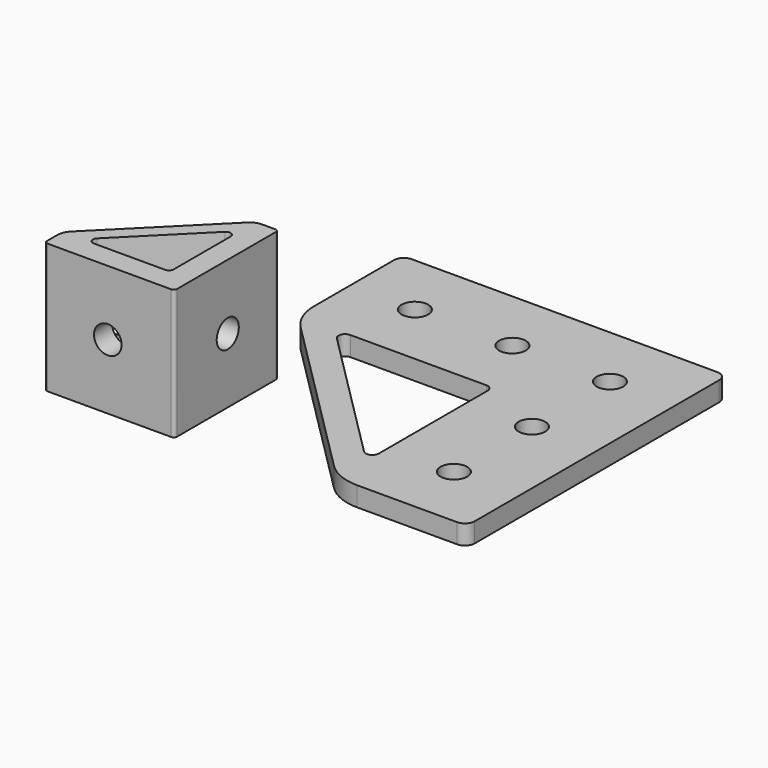
from build123d import *

# Parameters (mm, degrees)
F0_R           = 4.1
F1_DEPTH       = 6
F2_DEPTH       = 40
F5_D           = 8.5
F5_DEPTH       = 28
F5_TIP         = 2.5536576309
F5_ON_F3_D     = 8.5
F5_ON_F3_DEPTH = 28
F5_ON_F3_TIP   = 2.5536576309
F6_W           = 30
F6_H           = 20
F7_DEPTH       = 5
F8_R           = 9.99999
F9_R           = 5
F10_R          = 1.5
F11_R          = 1
F12_R          = 15
F13_R          = 2
F14_R          = 3


# Not quite as in the source:
# - a fillet or chamfer is up to 0.001 mm smaller than in the source, because OpenCascade refuses the exact size


with BuildPart() as f1:
    # F0 (on Top) → F1 (new body)
    with BuildSketch(Plane.XY):
        Polygon((78.5006253216, -80), (78.5006253216, 20), (-21.4993746784, 20), (-21.4993746784, -20), (-10.1856661794, -20), (38.5006253216, -20), (38.5006253216, -68.686291501), (38.5006253216, -80), align=None)
        with Locations((58.5006253216, -60)):
            Circle(F0_R, mode=Mode.SUBTRACT)
        with Locations((58.5006253216, -30)):
            Circle(F0_R, mode=Mode.SUBTRACT)
        with Locations((-1.4993746784, 0)):
            Circle(F0_R, mode=Mode.SUBTRACT)
        with Locations((28.5006253216, 0)):
            Circle(F0_R, mode=Mode.SUBTRACT)
        with Locations((58.5006253216, 0)):
            Circle(F0_R, mode=Mode.SUBTRACT)
        Polygon((-10.1856661794, -20), (-21.4993746784, -20), (38.5006253216, -80), (38.5006253216, -68.686291501), align=None)
    extrude(amount=F1_DEPTH)

    # F12
    f12_edges = [f1.edges().sort_by_distance(p)[0] for p in [
        (38.500625, -80, 3),
        (-21.499375, -20, 3),
    ]]
    fillet(f12_edges, radius=F12_R)

    # F13
    f13_edges = [f1.edges().sort_by_distance(p)[0] for p in [
        (38.500625, -20, 3),
        (-10.185666, -20, 3),
        (38.500625, -68.686292, 3),
    ]]
    fillet(f13_edges, radius=F13_R)

    # F14
    f14_edges = [f1.edges().sort_by_distance(p)[0] for p in [
        (-21.499375, 20, 3),
        (78.500625, 20, 3),
        (78.500625, -80, 3),
    ]]
    fillet(f14_edges, radius=F14_R)


with BuildPart() as f2:
    # F0 (on Top) → F2 (new body)
    with BuildSketch(Plane.XY):
        Polygon((-100, -19.3125), (-60, -19.3125), (-60, 20.6875), (-61, 20.6875), (-67, 14.6875), (-67, -12.3125), (-94, -12.3125), (-100, -18.3125), align=None)
        Polygon((-100, -12.3125), (-100, -18.3125), (-94, -12.3125), align=None)
        Polygon((-67, 20.6875), (-100, -12.3125), (-94, -12.3125), (-67, 14.6875), align=None)
        Polygon((-67, 14.6875), (-61, 20.6875), (-67, 20.6875), align=None)
    extrude(amount=-F2_DEPTH)

    # F5 (one way)
    with BuildSketch(Plane(origin=(-67, 0, 0), x_dir=(0, -1, 0), z_dir=(-1, 0, 0))):
        with Locations((-1.1875, -20)):
            Circle(F5_D / 2)
    extrude(amount=-F5_DEPTH, mode=Mode.SUBTRACT)
    with Locations(Plane(origin=(-67, 0, 0), x_dir=(0, -1, 0), z_dir=(-1, 0, 0))):
        with Locations((-1.1875, -20)):
            with Locations((0, 0, -(F5_DEPTH + F5_TIP / 2))):  # 118° drill point
                Cone(0, F5_D / 2, F5_TIP, mode=Mode.SUBTRACT)

    # F5 on F3 (one way)
    with BuildSketch(Plane(origin=(0, -12.3125, 0), x_dir=(-1, 0, 0), z_dir=(0, 1, 0))):
        with Locations((80.5, -20)):
            Circle(F5_ON_F3_D / 2)
    extrude(amount=-F5_ON_F3_DEPTH, mode=Mode.SUBTRACT)
    with Locations(Plane(origin=(0, -12.3125, 0), x_dir=(-1, 0, 0), z_dir=(0, 1, 0))):
        with Locations((80.5, -20)):
            with Locations((0, 0, -(F5_ON_F3_DEPTH + F5_ON_F3_TIP / 2))):  # 118° drill point
                Cone(0, F5_ON_F3_D / 2, F5_ON_F3_TIP, mode=Mode.SUBTRACT)

    # F6 (on face) → F7 (cut)
    with BuildSketch(Plane(origin=(-43.84375, 43.84375, 0), x_dir=(-0.7071067812, -0.7071067812, 0), z_dir=(-0.7071067812, 0.7071067812, 0))):
        with Locations((56.0478828037, -20)):
            Rectangle(F6_W, F6_H)
    extrude(amount=-F7_DEPTH, mode=Mode.SUBTRACT)

    # F8 (radius 10 in the source; OpenCascade refuses exactly that, so slightly less here)
    f8_edges = [f2.edges().sort_by_distance(p)[0] for p in [
        (-92.58219, -7.89469, -10),
        (-92.58219, -7.89469, -30),
        (-71.368986, 13.318514, -30),
        (-71.368986, 13.318514, -10),
    ]]
    fillet(f8_edges, radius=F8_R)

    # F9
    f9_edges = [f2.edges().sort_by_distance(p)[0] for p in [
        (-67, 20.6875, -20),
        (-100, -12.3125, -20),
    ]]
    fillet(f9_edges, radius=F9_R)

    # F10
    f10_edges = [f2.edges().sort_by_distance(p)[0] for p in [
        (-67, 14.6875, -20),
        (-67, -12.3125, -20),
        (-94, -12.3125, -20),
    ]]
    fillet(f10_edges, radius=F10_R)

    # F11
    f11_edges = [f2.edges().sort_by_distance(p)[0] for p in [
        (-60, 20.6875, -20),
        (-100, -19.3125, -20),
        (-60, -19.3125, -20),
    ]]
    fillet(f11_edges, radius=F11_R)


solid = Compound([f1.part, f2.part])
